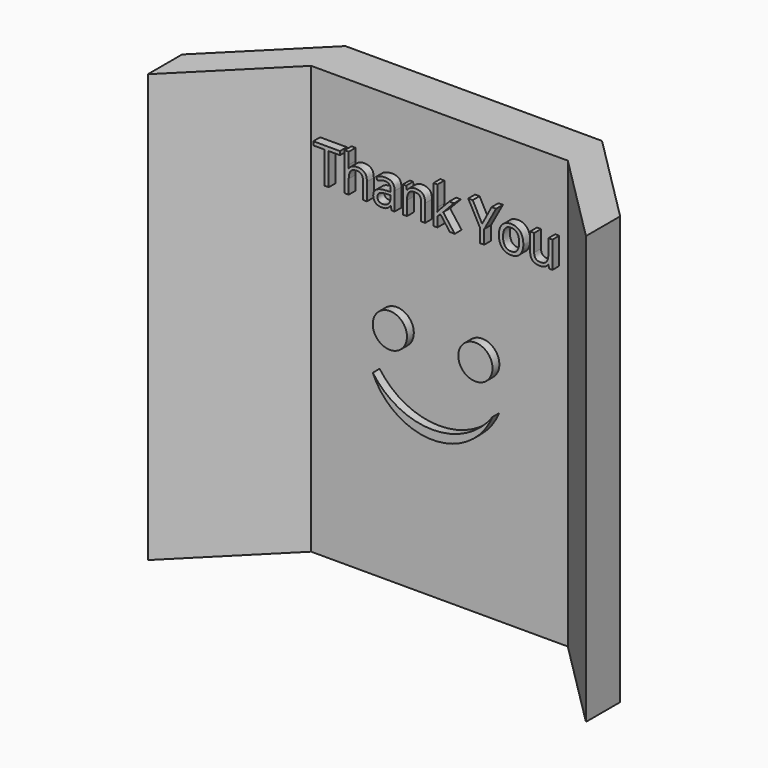
from build123d import *

# Parameters (mm, degrees)
F1_DEPTH     = 50
F2_R         = 2
F2_TEXT_SIZE = 5.8170486269
F3_DEPTH     = 1


# Not quite as in the source:
# - Text() gives the source's letters only with a copy of the font that has no kerning and outlines rounded to 1/6400 em; it was checked with that copy


with BuildPart() as f1:
    # F0 (on Top) → F1 (new body)
    with BuildSketch(Plane.XY):
        Polygon((-22.3804295258, 5.1419757109), (-22.3804295258, 0.1419757109), (-11.773827808, 10.7485774287), (18.226172192, 10.7485774287), (28.8327739098, 0.1419757109), (28.8327739098, 5.1419757109), (18.226172192, 15.7485774287), (-11.773827808, 15.7485774287), align=None)
    extrude(amount=F1_DEPTH)

    # F2 (on face) → F3 (join)
    with BuildSketch(Plane.XZ.offset(-10.7485774287)):
        with Locations((-1.773827808, 26.4290221306)):
            Circle(F2_R)
        with Locations((8.226172192, 26.4290221306)):
            Circle(F2_R)
        with BuildLine():
            ThreePointArc((10.226172192, 21.4290221306), (3.226172192, 17.8302957161), (-3.773827808, 21.4290221306))
            ThreePointArc((-3.773827808, 21.4290221306), (3.226172192, 16.7828039113), (10.226172192, 21.4290221306))
        make_face()
        with Locations((-10.773827808, 38.8359399279)):
            Text('Thank You', F2_TEXT_SIZE, font='Open Sans', text_align=(TextAlign.LEFT, TextAlign.BOTTOM))
    extrude(amount=F3_DEPTH)


solid = f1.part
